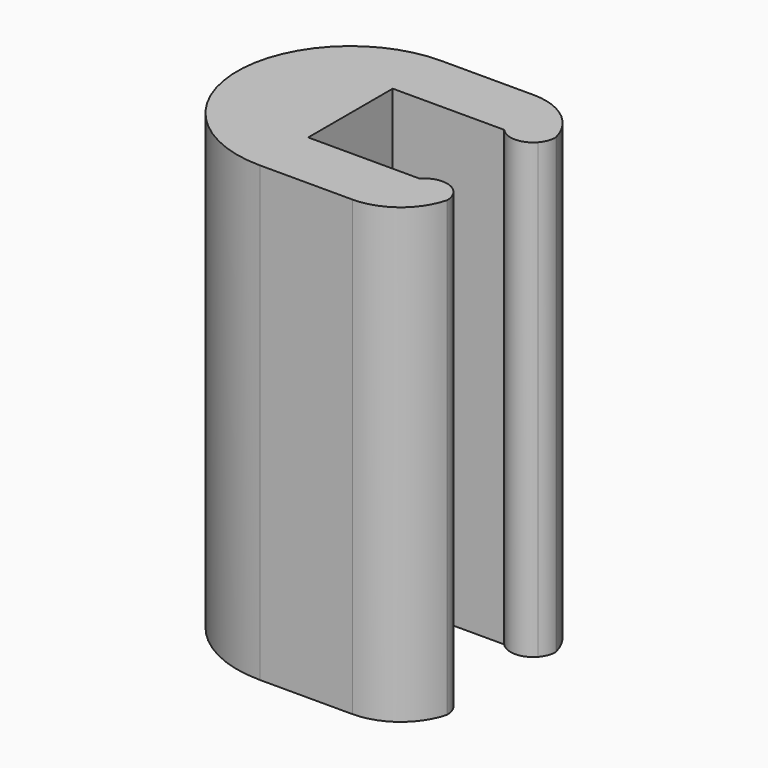
from build123d import *

# Parameters (mm, degrees)
F1_DEPTH    = 15
F2_T1_DEPTH = 24.6824583655


# Not quite as in the source:
# - a fillet or chamfer that OpenCascade refuses, or shapes differently, is made with other operations: its cross-section is extruded or revolved along the edge and cut away or added


with BuildPart() as f1:
    # F0 (on Top) → F1 (new body)
    with BuildSketch(Plane.XY):
        with BuildLine():
            Line((-5, 1.6397937215), (-1.6833752096, 1.6397937215))
            ThreePointArc((-1.6833752096, 1.6397937215), (-3.0635083269, 3.1011018661), (-5, 3.6397937215))
            ThreePointArc((-5, 3.6397937215), (-8.75, -0.1102062785), (-5, -3.8602062785))
            ThreePointArc((-5, -3.8602062785), (-3.0635083269, -3.3215144232), (-1.6833752096, -1.8602062785))
            Line((-1.6833752096, -1.8602062785), (-5, -1.8602062785))
            Line((-5, -1.8602062785), (-5, 1.6397937215))
        make_face()
        with BuildLine():
            ThreePointArc((-1.6833752096, -1.8602062785), (-3.0635083269, -3.3215144232), (-5, -3.8602062785))
            Line((-5, -3.8602062785), (0, -3.8602062785))
            Line((0, -3.8602062785), (0, -2.3602062785))
            ThreePointArc((0, -2.3602062785), (-1.0176165673, -3.0608355477), (-1.3090169944, -1.8602062785))
            Line((-1.3090169944, -1.8602062785), (-1.6833752096, -1.8602062785))
        make_face()
        with BuildLine():
            Line((-0.1909830056, -1.8602062785), (-1.3090169944, -1.8602062785))
            ThreePointArc((-1.3090169944, -1.8602062785), (-1.0176165673, -3.0608355477), (0, -2.3602062785))
            ThreePointArc((0, -2.3602062785), (-0.0493707308, -2.0925897112), (-0.1909830056, -1.8602062785))
        make_face()
        with BuildLine():
            ThreePointArc((-0.1909830056, -1.8602062785), (-0.75, -1.6102062785), (-1.3090169944, -1.8602062785))
            Line((-1.3090169944, -1.8602062785), (-0.1909830056, -1.8602062785))
        make_face()
        with BuildLine():
            ThreePointArc((-1.3090169944, 1.6397937215), (-0.75, 1.3897937215), (-0.1909830056, 1.6397937215))
            Line((-0.1909830056, 1.6397937215), (-1.3090169944, 1.6397937215))
        make_face()
        with BuildLine():
            Line((-1.3090169944, 1.6397937215), (-0.1909830056, 1.6397937215))
            ThreePointArc((-0.1909830056, 1.6397937215), (-0.0493707308, 1.8721771542), (0, 2.1397937215))
            ThreePointArc((0, 2.1397937215), (-1.0176165673, 2.8404229907), (-1.3090169944, 1.6397937215))
        make_face()
        with BuildLine():
            ThreePointArc((-1.3090169944, 1.6397937215), (-1.0176165673, 2.8404229907), (0, 2.1397937215))
            Line((0, 2.1397937215), (0, 3.6397937215))
            Line((0, 3.6397937215), (-5, 3.6397937215))
            ThreePointArc((-5, 3.6397937215), (-3.0635083269, 3.1011018661), (-1.6833752096, 1.6397937215))
            Line((-1.6833752096, 1.6397937215), (-1.3090169944, 1.6397937215))
        make_face()
    extrude(amount=F1_DEPTH)

    # F2: fillet of radius 2 on 2 edges, made by hand

    # F2_s2 → F2_t1 (cut)
    with BuildSketch(Plane.XY.offset(-4.8412291828)):
        with BuildLine():
            ThreePointArc((0, 2.1397937215), (-0.7117468017, 3.2209325516), (-1.9364916731, 3.6397937215))
            Line((-1.9364916731, 3.6397937215), (0, 3.6397937215))
            Line((0, 3.6397937215), (0, 2.1397937215))
        make_face()
        with BuildLine():
            ThreePointArc((-1.9364916731, -3.8602062785), (-0.7117468017, -3.4413451086), (0, -2.3602062785))
            Line((0, -2.3602062785), (0, -3.8602062785))
            Line((0, -3.8602062785), (-1.9364916731, -3.8602062785))
        make_face()
    extrude(amount=F2_T1_DEPTH, mode=Mode.SUBTRACT)


solid = f1.part
